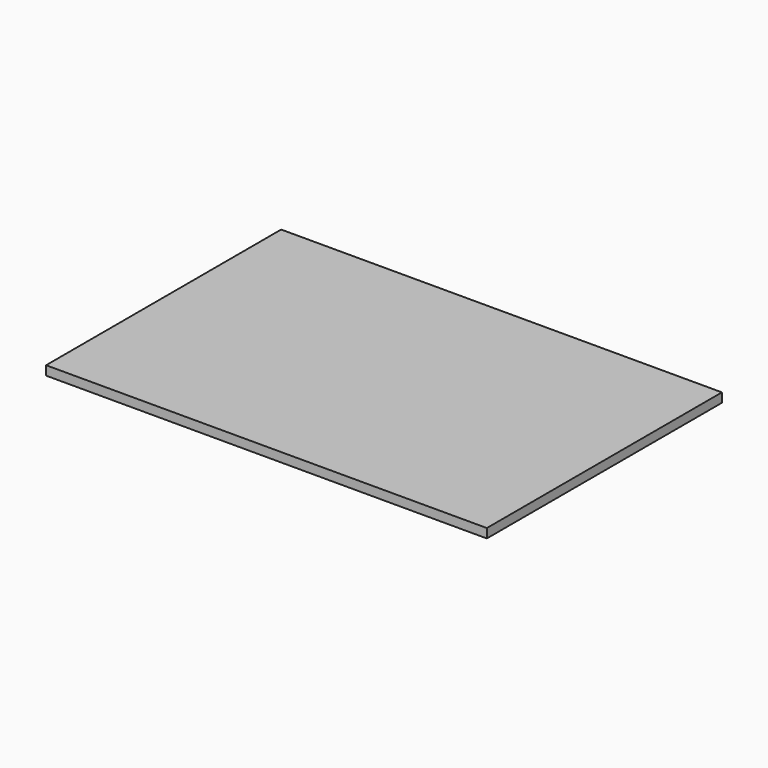
from build123d import *

# Parameters (mm, degrees)
F0_W     = 304.8
F0_H     = 203.2
F1_DEPTH = 6.35


# Not quite as in the source:
# - a length typed as a fraction of an inch, garbled in the dataset ("3 / 203.2 mm" for 3/8 in), is restored


with BuildPart() as f1:
    # F0 (on Top) → F1 (new body)
    with BuildSketch(Plane.XY):
        Rectangle(F0_W, F0_H)
    extrude(amount=F1_DEPTH)


solid = f1.part
